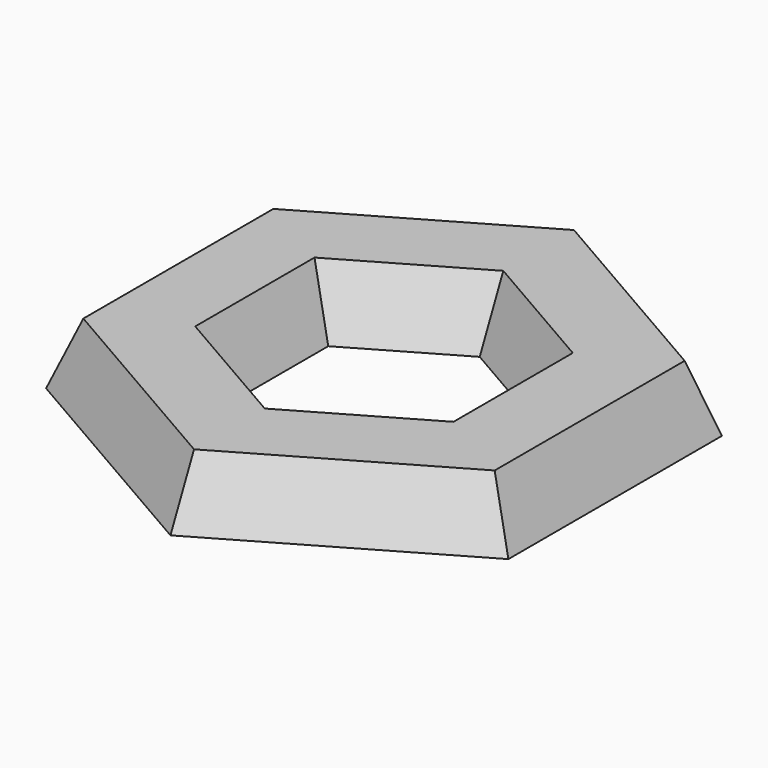
from build123d import *

# Parameters (mm, degrees)
F1_DEPTH = 2
F2_SIZE2 = 0.79999
F2_SIZE  = 1.99999


# Not quite as in the source:
# - a fillet or chamfer is up to 0.001 mm smaller than in the source, because OpenCascade refuses the exact size


with BuildPart() as f1:
    # F0 (on Top) → F1 (new body)
    with BuildSketch(Plane.XY):
        Polygon((-7.25, 4.1857894516), (-7.25, -4.1857894516), (0, -8.3715789032), (7.25, -4.1857894516), (7.25, 4.1857894516), (0, 8.3715789032), align=None)
        Polygon((0, 3.7527767497), (3.25, 1.8763883749), (3.25, -1.8763883749), (0, -3.7527767497), (-3.25, -1.8763883749), (-3.25, 1.8763883749), align=None, mode=Mode.SUBTRACT)
    extrude(amount=F1_DEPTH)

    # F2 (size 2 and 0.8 in the source; OpenCascade refuses exactly that, so slightly less here)
    f2_edges = [f1.edges().sort_by_distance(p)[0] for p in [
        (-7.25, 0, 2),
        (-3.625, -6.278684, 2),
        (3.625, -6.278684, 2),
        (7.25, 0, 2),
        (3.625, 6.278684, 2),
        (-3.625, 6.278684, 2),
        (-3.25, 0, 2),
        (-1.625, 2.814583, 2),
        (1.625, 2.814583, 2),
        (3.25, 0, 2),
        (1.625, -2.814583, 2),
        (-1.625, -2.814583, 2),
    ]]
    chamfer(f2_edges, length=F2_SIZE, length2=F2_SIZE2)


solid = f1.part
